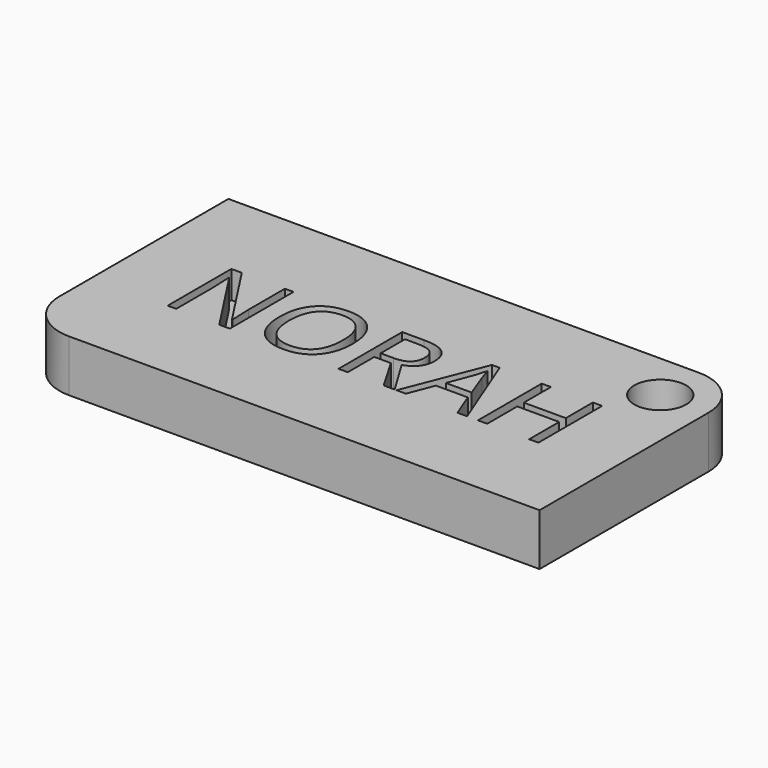
from build123d import *

# Parameters (mm, degrees)
F0_W         = 50.8
F0_H         = 25.4
F1_DEPTH     = 5.08
F2_TEXT_SIZE = 10.921306042
F3_DEPTH     = 2.6924
F4_R         = 4.7217188853
F5_R         = 2.54
F6_DEPTH     = 5.081


# Not quite as in the source:
# - Text() gives the source's letters only with a copy of the font that has no kerning and outlines rounded to 1/6400 em; it was checked with that copy


with BuildPart() as f1:
    # F0 (on Top) → F1 (new body)
    with BuildSketch(Plane.XY):
        Rectangle(F0_W, F0_H)
    extrude(amount=F1_DEPTH)

    # F2 (on face) → F3 (cut)
    with BuildSketch(Plane.XY.offset(5.08)):
        with Locations((-19.05, -4.0165465591)):
            Text('NORAH', F2_TEXT_SIZE, font='Open Sans', text_align=(TextAlign.LEFT, TextAlign.BOTTOM))
    extrude(amount=-F3_DEPTH, mode=Mode.SUBTRACT)

    # F4
    f4_edges = [f1.edges().sort_by_distance(p)[0] for p in [
        (25.4, 12.7, 2.54),
        (-25.4, -12.7, 2.54),
    ]]
    fillet(f4_edges, radius=F4_R)

    # F5 (on face) → F6 (cut, through all)
    with BuildSketch(Plane.XY.offset(5.08)):
        with Locations((20.6782811147, 7.9782811147)):
            Circle(F5_R)
    extrude(amount=-F6_DEPTH, mode=Mode.SUBTRACT)


solid = f1.part
